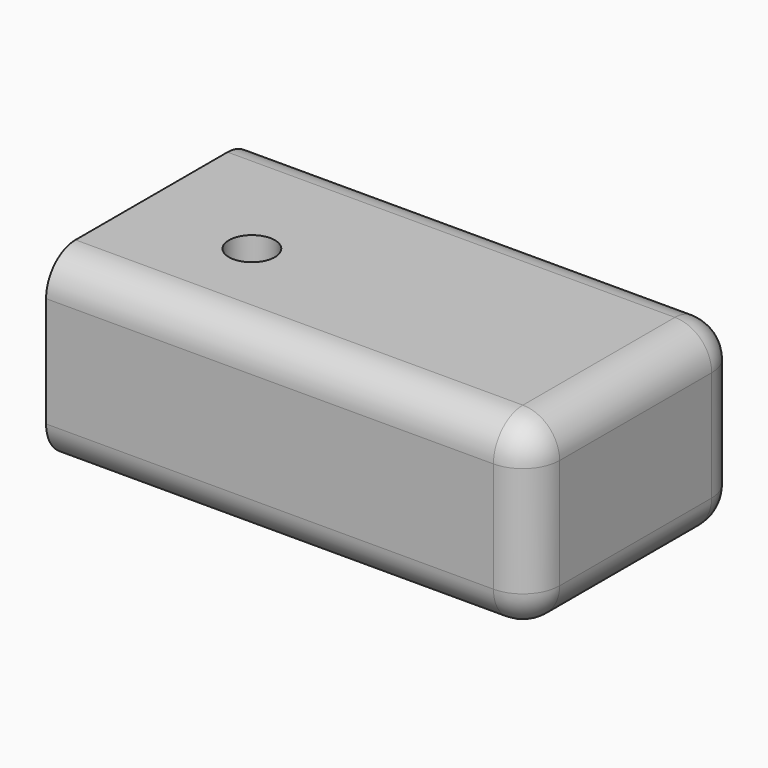
from build123d import *

# Parameters (mm, degrees)
F0_W     = 66.9010188431
F0_H     = 36.4210186526
F1_DEPTH = 25.4
F2_R     = 5.08
F3_R     = 5.08
F4_R     = 5.08
F5_R     = 5.08
F6_R     = 5.08
F7_T     = 5.08
F9_D     = 6.35


# Not quite as in the source:
# - a shell that OpenCascade refuses in one call is made with other operations: the cavity is built on its own and cut out


with BuildPart() as f1:
    # F0 (on Top) → F1 (new body)
    with BuildSketch(Plane.XY):
        with Locations((6.1347456649, -7.5554237701)):
            Rectangle(F0_W, F0_H)
    extrude(amount=F1_DEPTH)

    # F2
    f2_edges = [f1.edges().sort_by_distance(p)[0] for p in [
        (6.134746, 10.655086, 25.4),
    ]]
    fillet(f2_edges, radius=F2_R)

    # F3
    f3_edges = [f1.edges().sort_by_distance(p)[0] for p in [
        (6.134746, 10.655086, 0),
    ]]
    fillet(f3_edges, radius=F3_R)

    # F4
    f4_edges = [f1.edges().sort_by_distance(p)[0] for p in [
        (6.134746, -25.765933, 25.4),
    ]]
    fillet(f4_edges, radius=F4_R)

    # F5
    f5_edges = [f1.edges().sort_by_distance(p)[0] for p in [
        (6.134746, -25.765933, 0),
    ]]
    fillet(f5_edges, radius=F5_R)

    # F6
    f6_edges = [f1.edges().sort_by_distance(p)[0] for p in [
        (39.585255, -7.555424, 0),
        (39.585255, 9.167188, 1.487898),
        (39.585255, 9.167188, 23.912102),
        (39.585255, 10.655086, 12.7),
        (39.585255, -7.555424, 25.4),
        (39.585255, -24.278036, 1.487898),
        (39.585255, -25.765933, 12.7),
        (39.585255, -24.278036, 23.912102),
    ]]
    fillet(f6_edges, radius=F6_R)

    # F7: shell of thickness 5.08, made by hand


with BuildPart() as f7_core1:
    # F7_t2: copy of F1
    add(f1.part)

    # the walls: a layer under each face that stays
    f7_faces = [f7_core1.faces().sort_by_distance(p)[0] for p in [
        (39.5852550864, -7.5554237701, 12.7),
        (3.5947456649, -7.5554237701, 0),
        (3.5947456649, -25.7659330964, 12.7),
        (3.5947456649, 10.6550855562, 12.7),
        (3.5947456649, -7.5554237701, 25.4),
    ]]
    thicken(f7_faces, amount=-F7_T, mode=Mode.SUBTRACT)


with BuildPart() as f1_1:
    add(f1.part)

    # what is left inside the walls is the cavity
    f7_cavity = [f7_core1.part.solids().sort_by_distance(p)[0] for p in [
        (3.594746, -11.93226, 5.1308),
    ]]
    add(f7_cavity, mode=Mode.SUBTRACT)

    # F9 (through all)
    with Locations(Plane(origin=(0, 0, 0), x_dir=(1, 0, 0), z_dir=(0, 0, -1))):
        with Locations((-11.171694845, 10.3967795148)):
            Hole(F9_D / 2)


solid = f1_1.part
